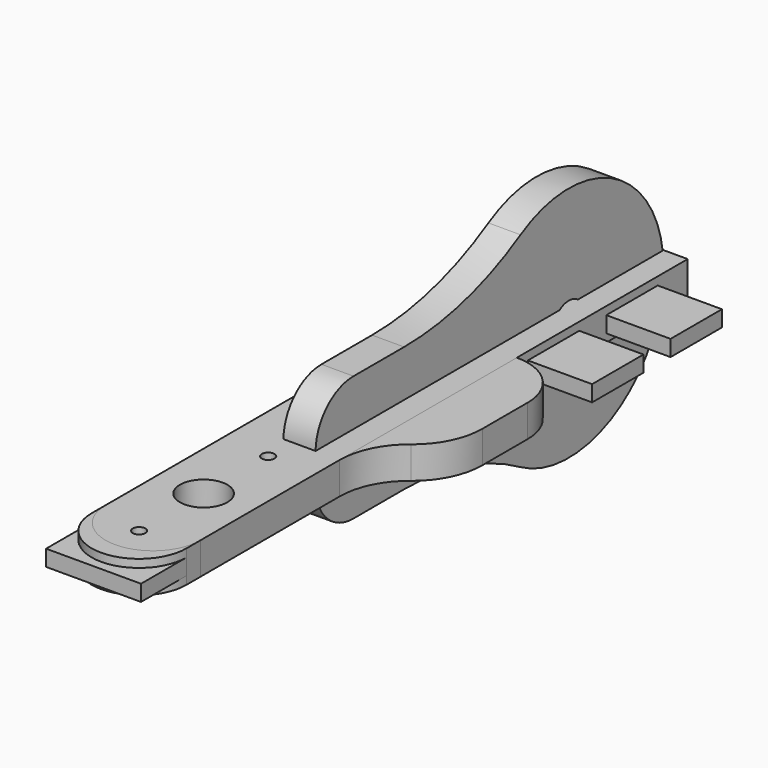
from build123d import *

# Parameters (mm, degrees)
F1_R      = 1.016
F1_R_2    = 3.81
F2_DEPTH  = 1.28905
F3_R      = 1.75
F3_R_2    = 3.81
F4_DEPTH  = 2.5781
F5_R      = 1.27
F6_R      = 6.34999
F9_R      = 3.175
F10_DEPTH = 2.5781
F11_R     = 1.27
F12_R     = 7.61999
F13_W     = 15.24
F13_H     = 105.41
F13_R     = 1.016
F13_R_2   = 3.81
F14_DEPTH = 2.5781
F15_R     = 7.61999


# Not quite as in the source:
# - a variable given as a bare number and used for a length is read in inches; the dataset says mm whatever the document's units were
# - a fillet or chamfer is up to 0.001 mm smaller than in the source, because OpenCascade refuses the exact size


with BuildPart() as f2:
    # F1 (on Top) → F2 (new body, symmetric)
    with BuildSketch(Plane.XY):
        Polygon((-7.62, 66.0019), (-7.62, -22.098), (7.62, -22.098), (7.62, 55.5498), (17.9324, 55.5498), (17.9324, 65.8622), (7.62, 65.8622), (7.62, 71.2978), (17.9324, 71.2978), (17.9324, 81.6102), (7.62, 81.6102), (-7.62, 81.6102), (-7.62, 71.1581), (-13.97, 71.1581), (-13.97, 66.0019), align=None)
        with Locations((0, -12.954)):
            Circle(F1_R, mode=Mode.SUBTRACT)
        Circle(F1_R_2, mode=Mode.SUBTRACT)
        with Locations((0, 12.954)):
            Circle(F1_R, mode=Mode.SUBTRACT)
    extrude(amount=F2_DEPTH, both=True)


with BuildPart() as f4:
    # F3 (on Top) → F4 (new body, symmetric)
    with BuildSketch(Plane.XY):
        with BuildLine():
            Line((7.62, -12.954), (7.62, 17.78))
            ThreePointArc((7.62, 17.78), (8.7639049612, 22.7271512904), (11.9634, 26.67))
            ThreePointArc((11.9634, 26.67), (15.1628950388, 30.6128487096), (16.3068, 35.56))
            Line((16.3068, 35.56), (16.3068, 44.6532))
            ThreePointArc((16.3068, 44.6532), (13.7624951868, 50.7956951868), (7.62, 53.34))
            Line((7.62, 53.34), (3.6068, 53.34))
            Line((3.6068, 53.34), (3.6068, 35.56))
            Line((3.6068, 35.56), (-1.27, 35.56))
            Line((-1.27, 35.56), (-1.27, 53.34))
            Line((-1.27, 53.34), (-7.62, 53.34))
            Line((-7.62, 53.34), (-7.62, -12.954))
            ThreePointArc((-7.62, -12.954), (0, -20.574), (7.62, -12.954))
        make_face()
        with Locations((0, -12.954)):
            Circle(F3_R, mode=Mode.SUBTRACT)
        Circle(F3_R_2, mode=Mode.SUBTRACT)
        with Locations((0, 12.954)):
            Circle(F3_R, mode=Mode.SUBTRACT)
    extrude(amount=F4_DEPTH, both=True)

    # F5
    f5_edges = [f4.edges().sort_by_distance(p)[0] for p in [
        (3.6068, 35.56, 0),
        (-1.27, 35.56, 0),
    ]]
    fillet(f5_edges, radius=F5_R)

    # F6 (radius 6.35 in the source; OpenCascade refuses exactly that, so slightly less here)
    f6_edges = [f4.edges().sort_by_distance(p)[0] for p in [
        (-7.62, 53.34, 0),
    ]]
    fillet(f6_edges, radius=F6_R)


with BuildPart() as f10:
    # F9 (on plane+point) → F10 (new body, symmetric)
    with BuildSketch(Plane.YZ.offset(1.1684)):
        with BuildLine():
            ThreePointArc((58.9212849333, -16.4198575895), (78.0379061631, -16.5363391054), (87.63, 0))
            ThreePointArc((87.63, 0), (78.0379061631, 16.5363391054), (58.9212849333, 16.4198575895))
            ThreePointArc((58.9212849333, 16.4198575895), (49.53, 0), (58.9212849333, -16.4198575895))
        make_face()
        with Locations((68.58, 0)):
            Circle(F9_R, mode=Mode.SUBTRACT)
        with BuildLine():
            ThreePointArc((58.9212849333, -16.4198575895), (49.53, 0), (58.9212849333, 16.4198575895))
            ThreePointArc((58.9212849333, 16.4198575895), (47.665967293, 11.6772014663), (35.56, 10.0584))
            Line((35.56, 10.0584), (17.78, 10.0584))
            Line((17.78, 10.0584), (17.78, 2.4384))
            Line((17.78, 2.4384), (35.56, 2.4384))
            Line((35.56, 2.4384), (35.56, 0))
            Line((35.56, 0), (35.56, -2.4384))
            Line((35.56, -2.4384), (17.78, -2.4384))
            Line((17.78, -2.4384), (17.78, -10.0584))
            Line((17.78, -10.0584), (35.56, -10.0584))
            ThreePointArc((35.56, -10.0584), (47.665967293, -11.6772014663), (58.9212849333, -16.4198575895))
        make_face()
    extrude(amount=F10_DEPTH, both=True)

    # F11
    f11_edges = [f10.edges().sort_by_distance(p)[0] for p in [
        (1.1684, 35.56, 2.4384),
        (1.1684, 35.56, -2.4384),
    ]]
    fillet(f11_edges, radius=F11_R)

    # F12 (radius 7.62 in the source; OpenCascade refuses exactly that, so slightly less here)
    f12_edges = [f10.edges().sort_by_distance(p)[0] for p in [
        (1.1684, 17.78, -10.0584),
        (1.1684, 17.78, 10.0584),
    ]]
    fillet(f12_edges, radius=F12_R)


with BuildPart() as f14:
    # F13 (on Top) → F14 (new body, symmetric)
    with BuildSketch(Plane.XY):
        with Locations((0, 34.925)):
            Rectangle(F13_W, F13_H)
        with Locations((0, -12.954)):
            Circle(F13_R, mode=Mode.SUBTRACT)
        Circle(F13_R_2, mode=Mode.SUBTRACT)
        with Locations((0, 12.954)):
            Circle(F13_R, mode=Mode.SUBTRACT)
    extrude(amount=F14_DEPTH, both=True)

    # F15 (radius 7.62 in the source; OpenCascade refuses exactly that, so slightly less here)
    f15_edges = [f14.edges().sort_by_distance(p)[0] for p in [
        (7.62, -17.78, 0),
        (-7.62, -17.78, 0),
    ]]
    fillet(f15_edges, radius=F15_R)


solid = Compound([f2.part, f4.part, f10.part, f14.part])
